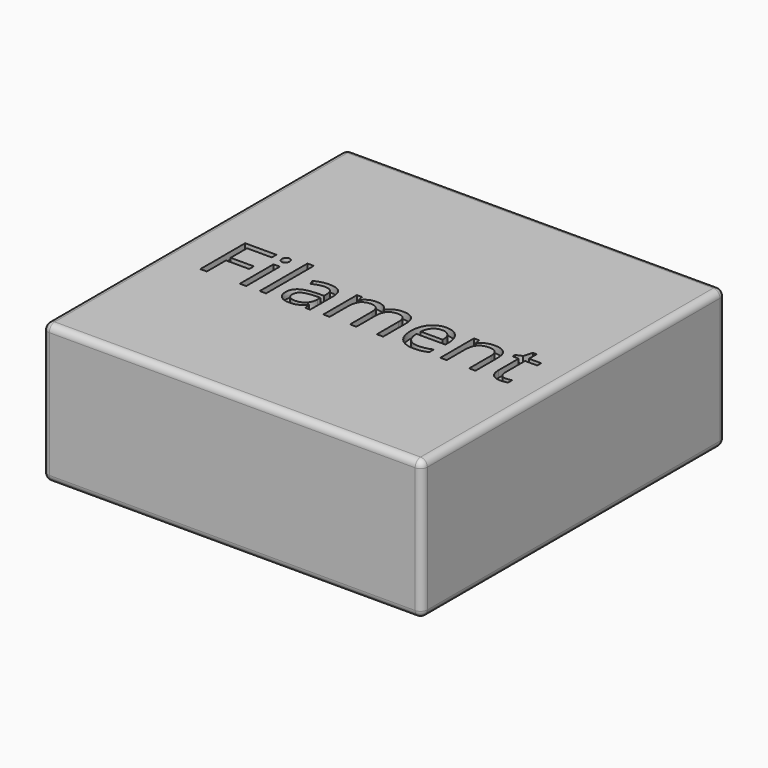
from build123d import *

# Parameters (mm, degrees)
F0_W         = 225
F0_H         = 225
F1_DEPTH     = 82.5
F2_R         = 4
F3_TEXT_SIZE = 46.568627451
F4_DEPTH     = 4


# Not quite as in the source:
# - Text() gives the source's letters only with a copy of the font that has no kerning and outlines rounded to 1/6400 em; it was checked with that copy


with BuildPart() as f1:
    # F0 (on Top) → F1 (new body)
    with BuildSketch(Plane.XY):
        with Locations((-112.5, 112.5)):
            Rectangle(F0_W, F0_H)
    extrude(amount=F1_DEPTH)

    # F2
    f2_edges = [f1.edges().sort_by_distance(p)[0] for p in [
        (-225, 0, 41.25),
        (0, 0, 41.25),
        (-112.5, 0, 0),
        (-112.5, 0, 82.5),
        (0, 225, 41.25),
        (0, 112.5, 0),
        (0, 112.5, 82.5),
        (-112.5, 225, 82.5),
        (-225, 112.5, 82.5),
        (-225, 225, 41.25),
        (-225, 112.5, 0),
        (-112.5, 225, 0),
    ]]
    fillet(f2_edges, radius=F2_R)

    # F3 (on face) → F4 (cut)
    with BuildSketch(Plane.XY.offset(82.5)):
        with Locations((-206, 87.4705882353)):
            Text('Filament', F3_TEXT_SIZE, font='Open Sans', text_align=(TextAlign.LEFT, TextAlign.BOTTOM))
    extrude(amount=-F4_DEPTH, mode=Mode.SUBTRACT)


solid = f1.part
